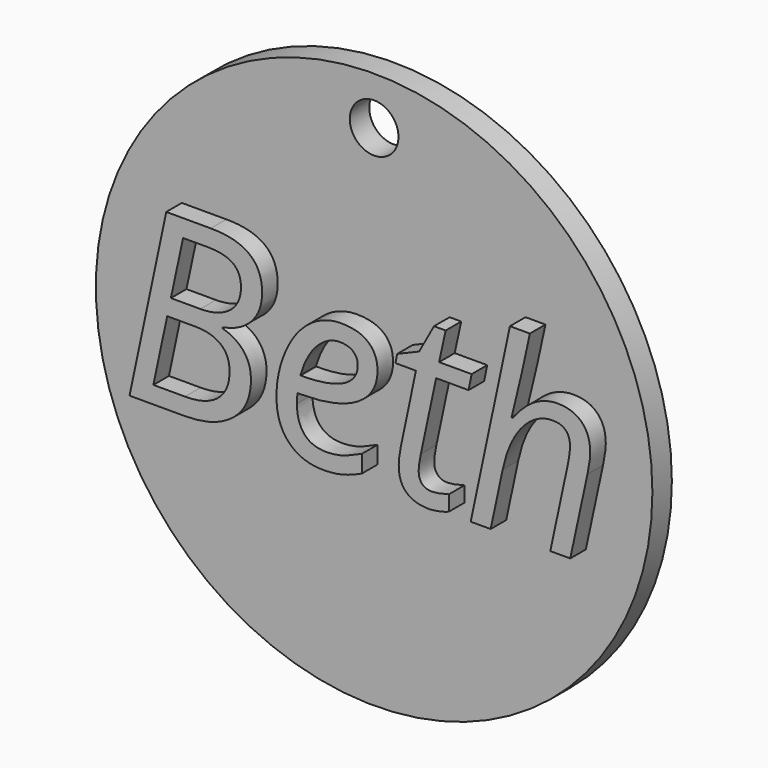
from build123d import *

# Parameters (mm, degrees)
F0_R         = 28.575
F1_DEPTH     = 1.25
F2_TEXT_SIZE = 24.9844794679
F3_DEPTH     = 2
F5_D         = 5


# Not quite as in the source:
# - Text() gives the source's letters only with a copy of the font that has no kerning and outlines rounded to 1/6400 em; it was checked with that copy


with BuildPart() as f1:
    # F0 (on Front) → F1 (new body, symmetric)
    with BuildSketch(Plane.XZ):
        Circle(F0_R)
    extrude(amount=F1_DEPTH, both=True)

    # F2 (on face) → F3 (join)
    with BuildSketch(Plane.XZ.offset(1.25)):
        with Locations((-24.5668292046, -7.3834732175)):
            Text('Beth', F2_TEXT_SIZE, font='Open Sans', font_style=FontStyle.ITALIC, text_align=(TextAlign.LEFT, TextAlign.BOTTOM))
    extrude(amount=F3_DEPTH)

    # F5 (through all)
    with Locations(Plane.XZ.offset(1.25)):
        with Locations((0, 23.651426658)):
            Hole(F5_D / 2)


solid = f1.part
